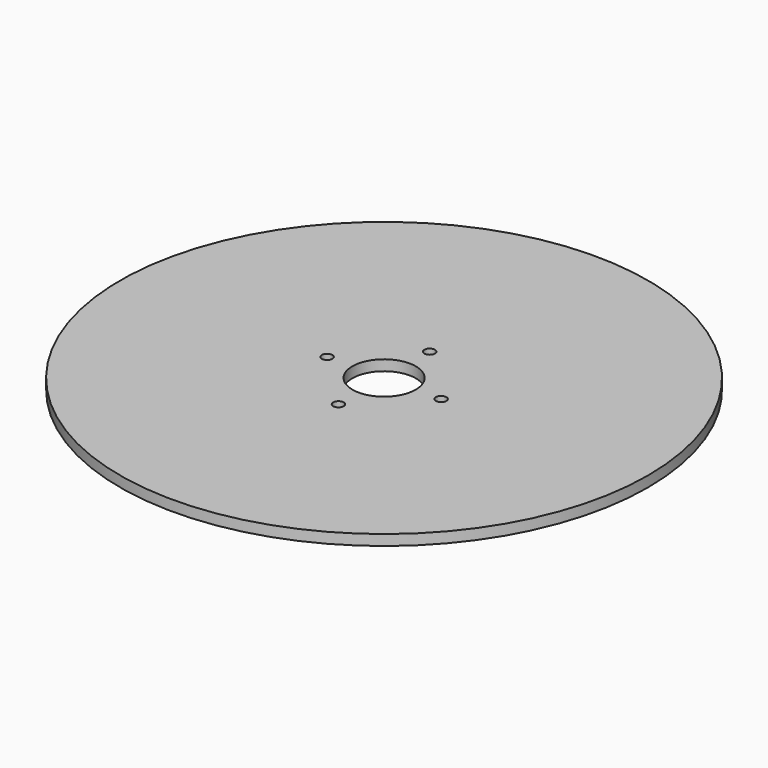
from build123d import *

# Parameters (mm, degrees)
F0_R            = 125
F2_DEPTH        = 5
F1_R            = 15
F3_DEPTH        = 5.001
F5_D            = 5
F5_COPIES_COUNT = 4


# Not quite as in the source:
# - a pattern or mirror of a feature is missing from the dataset's text; its kind, count and spacing are read off the source's solid
# - a feature names something its author has since deleted; it is built from what else it names


with BuildPart() as f2:
    # F0 (on Top) → F2 (new body)
    with BuildSketch(Plane.XY):
        Circle(F0_R)
    extrude(amount=F2_DEPTH)

    # F1 (on Top) → F3 (cut, through all)
    with BuildSketch(Plane.XY):
        Circle(F1_R)
    extrude(amount=F3_DEPTH, mode=Mode.SUBTRACT)

    # F5 (through all)
    with Locations(Plane(origin=(0, 0, 0), x_dir=(1, 0, 0), z_dir=(0, 0, -1))):
        with Locations((0, -27)):
            f5 = Hole(F5_D / 2)

    # F5_copies: F5 ×4 about axis
    f5_copies_axis = Axis((0, 0, 0), (0, 0, 1))
    for i in range(1, F5_COPIES_COUNT):
        add(f5.rotate(f5_copies_axis, i * 360 / F5_COPIES_COUNT), mode=Mode.SUBTRACT)


solid = f2.part
